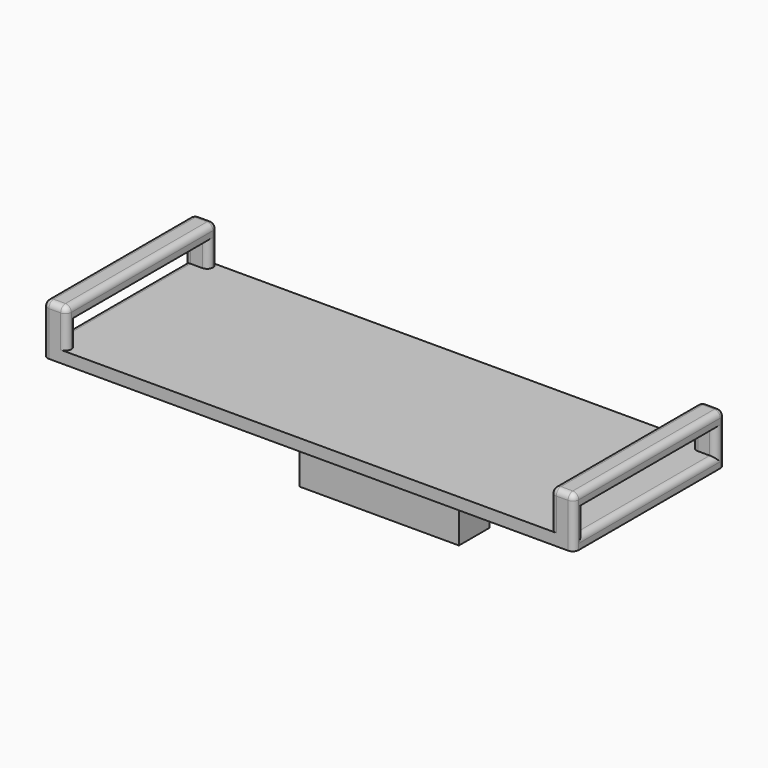
from build123d import *

# Parameters (mm, degrees)
F0_W      = 90
F0_H      = 32
F1_DEPTH  = 2
F2_W      = 4
F2_H      = 2
F3_DEPTH  = 6.5
F5_W      = 4
F5_H      = 2
F6_DEPTH  = 28
F4_W      = 4
F4_H      = 2
F7_DEPTH  = 28
F8_R      = 0.99999
F10_DEPTH = 15.25


# Not quite as in the source:
# - a fillet or chamfer is up to 0.001 mm smaller than in the source, because OpenCascade refuses the exact size


with BuildPart() as f1:
    # F0 (on Top) → F1 (new body)
    with BuildSketch(Plane.XY):
        with Locations((45, 16)):
            Rectangle(F0_W, F0_H)
    extrude(amount=F1_DEPTH)

    # F2 (on face) → F3 (join)
    with BuildSketch(Plane.XY.offset(2)):
        with Locations((2, 31)):
            Rectangle(F2_W, F2_H)
        with Locations((2, 1)):
            Rectangle(F2_W, F2_H)
        with Locations((88, 1)):
            Rectangle(F2_W, F2_H)
        with Locations((88, 31)):
            Rectangle(F2_W, F2_H)
    extrude(amount=F3_DEPTH)

    # F5 (on face) → F6 (join)
    with BuildSketch(Plane(origin=(0, 2, 0), x_dir=(-1, 0, 0), z_dir=(0, 1, 0))):
        with Locations((-2, 7.5)):
            Rectangle(F5_W, F5_H)
    extrude(amount=F6_DEPTH)

    # F4 (on face) → F7 (join)
    with BuildSketch(Plane(origin=(0, 2, 0), x_dir=(-1, 0, 0), z_dir=(0, 1, 0))):
        with Locations((-88, 7.5)):
            Rectangle(F4_W, F4_H)
    extrude(amount=F7_DEPTH)

    # F8 (radius 1 in the source; OpenCascade refuses exactly that, so slightly less here)
    f8_edges = [f1.edges().sort_by_distance(p)[0] for p in [
        (0, 16, 8.5),
        (4, 16, 8.5),
        (0, 32, 4.25),
        (0, 0, 4.25),
        (0, 16, 2),
        (2, 32, 8.5),
        (2, 0, 8.5),
        (0, 30, 4.25),
        (0, 2, 4.25),
        (4, 2, 4.25),
        (4, 30, 4.25),
        (4, 32, 5.25),
        (4, 0, 5.25),
        (86, 0, 5.25),
        (90, 0, 4.25),
        (86, 30, 4.25),
        (90, 30, 4.25),
        (86, 32, 5.25),
        (90, 32, 4.25),
        (90, 16, 8.5),
        (86, 16, 8.5),
        (88, 0, 8.5),
        (88, 32, 8.5),
        (90, 2, 4.25),
        (90, 16, 2),
    ]]
    fillet(f8_edges, radius=F8_R)

    # F9 (on face) → F10 (join)
    with BuildSketch(Plane(origin=(0, 0, 0), x_dir=(1, 0, 0), z_dir=(0, 0, -1))):
        Polygon((33.5, -30), (33.5, -25.5), (31.5, -25.5), (31.5, -32), (58.5, -32), (58.5, -25.5), (56.5, -25.5), (56.5, -30), align=None)
        Polygon((33.5, -21.5), (33.5, -17), (56.5, -17), (56.5, -21.5), (58.5, -21.5), (58.5, -15), (31.5, -15), (31.5, -21.5), align=None)
    extrude(amount=F10_DEPTH)


solid = f1.part
